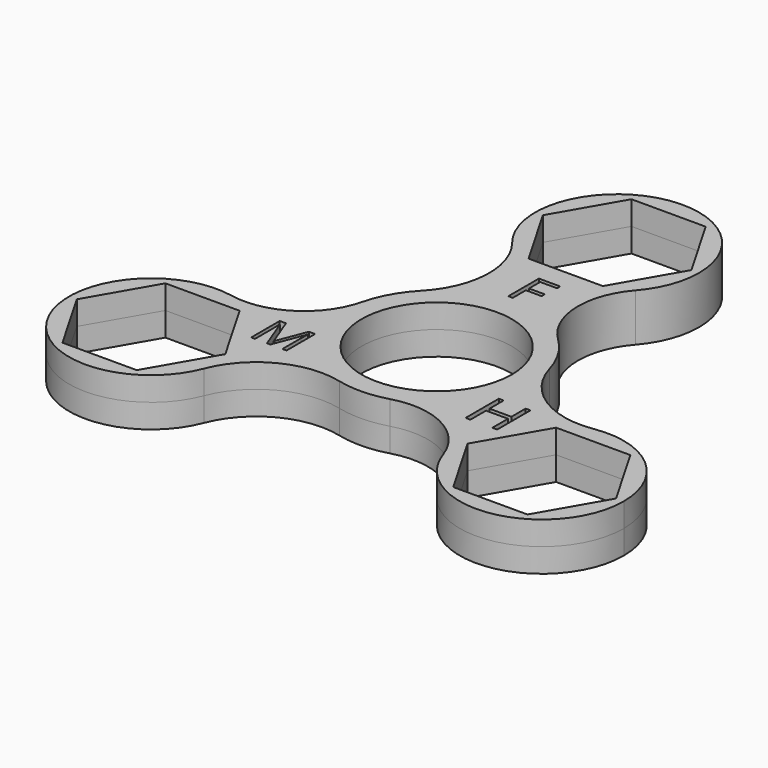
from build123d import *

# Parameters (mm, degrees)
F0_R           = 11
F1_DEPTH       = 3.5
F2_TEXT_SIZE   = 7.8320322144
F2_TEXT_SIZE_2 = 7.3181788644
F2_TEXT_SIZE_3 = 8.5313190033
F3_DEPTH       = 25


# Not quite as in the source:
# - Text() gives the source's letters only with a copy of the font that has no kerning and outlines rounded to 1/6400 em; it was checked with that copy


with BuildPart() as f1:
    # F0 (on Top) → F1 (new body, symmetric)
    with BuildSketch(Plane.XY):
        with BuildLine():
            ThreePointArc((-10.0686173445, 9.7274325889), (-0.2691708914, 13.9974121548), (9.6871937816, 10.1073377621))
            ThreePointArc((9.6871937816, 10.1073377621), (6.347333438, 17.4828570683), (9.0292648557, 25.1222415999))
            ThreePointArc((9.0292648557, 25.1222415999), (-0.2504407288, 21.0288021139), (-9.3512391392, 25.5059274026))
            ThreePointArc((-9.3512391392, 25.5059274026), (-6.7280894472, 17.4811090057), (-10.0686173445, 9.7274325889))
        make_face()
        with BuildLine():
            ThreePointArc((3.9096143758, -13.4430247873), (11.1967540221, -8.4043262293), (14, 0))
            ThreePointArc((14, 0), (13.863967212, 1.9468983398), (13.4585124078, 3.8559621069))
            ThreePointArc((13.4585124078, 3.8559621069), (11.9875290676, 7.2318149073), (9.6871937816, 10.1073377621))
            ThreePointArc((9.6871937816, 10.1073377621), (-0.2691708914, 13.9974121548), (-10.0686173445, 9.7274325889))
            ThreePointArc((-10.0686173445, 9.7274325889), (-12.256699959, 6.7655972475), (-13.5968081574, 3.3356870252))
            ThreePointArc((-13.5968081574, 3.3356870252), (-11.9875290676, -7.2318149073), (-3.3898950633, -13.5833946957))
            ThreePointArc((-3.3898950633, -13.5833946957), (0.2691708914, -13.9974121548), (3.9096143758, -13.4430247873))
        make_face()
        Circle(F0_R, mode=Mode.SUBTRACT)
        with BuildLine():
            ThreePointArc((-17.4131615082, -20.8513743528), (-11.7750397617, -14.567250883), (-3.3898950633, -13.5833946957))
            ThreePointArc((-3.3898950633, -13.5833946957), (-11.9875290676, -7.2318149073), (-13.5968081574, 3.3356870252))
            ThreePointArc((-13.5968081574, 3.3356870252), (-18.3142650709, -3.2444765306), (-26.2711318534, -4.7415480575))
            ThreePointArc((-26.2711318534, -4.7415480575), (-19.3288531038, -8.8961603469), (-16.6015182075, -16.5130942363))
            ThreePointArc((-16.6015182075, -16.5130942363), (-16.8061742025, -18.7198701207), (-17.4131615082, -20.8513743528))
        make_face()
        with BuildLine():
            ThreePointArc((13.4585124078, 3.8559621069), (13.863967212, 1.9468983398), (14, 0))
            ThreePointArc((14, 0), (11.1967540221, -8.4043262293), (3.9096143758, -13.4430247873))
            ThreePointArc((3.9096143758, -13.4430247873), (11.9669316329, -14.2383805377), (17.2418669977, -20.3806935425))
            ThreePointArc((17.2418669977, -20.3806935425), (18.3366972061, -10.2975130237), (26.7644006474, -4.6545530499))
            ThreePointArc((26.7644006474, -4.6545530499), (18.5031292089, -2.9138581227), (13.4585124078, 3.8559621069))
        make_face()
        with BuildLine():
            ThreePointArc((-9.3512391392, 25.5059274026), (-0.2504407288, 21.0288021139), (9.0292648557, 25.1222415999))
            ThreePointArc((9.0292648557, 25.1222415999), (11.232790799, 28.8042918768), (12, 33.0261884726))
            ThreePointArc((12, 33.0261884726), (-3.9865480261, 44.3446439695), (-9.3512391392, 25.5059274026))
        make_face()
        Polygon((10.8715055688, 33.0261884726), (5.4357527844, 23.6111884726), (-5.4357527844, 23.6111884726), (-10.8715055688, 33.0261884726), (-5.4357527844, 42.4411884726), (5.4357527844, 42.4411884726), align=None, mode=Mode.SUBTRACT)
        with BuildLine():
            ThreePointArc((-26.2711318534, -4.7415480575), (-39.1167799376, -22.2948993824), (-17.4131615082, -20.8513743528))
            ThreePointArc((-17.4131615082, -20.8513743528), (-16.8061742025, -18.7198701207), (-16.6015182075, -16.5130942363))
            ThreePointArc((-16.6015182075, -16.5130942363), (-19.3288531038, -8.8961603469), (-26.2711318534, -4.7415480575))
        make_face()
        Polygon((-23.1657654231, -25.9280942363), (-34.0372709919, -25.9280942363), (-39.4730237763, -16.5130942363), (-34.0372709919, -7.0980942363), (-23.1657654231, -7.0980942363), (-17.7300126386, -16.5130942363), align=None, mode=Mode.SUBTRACT)
        with BuildLine():
            ThreePointArc((40.6015182075, -16.5130942363), (36.4103141863, -7.4014146238), (26.7644006474, -4.6545530499))
            ThreePointArc((26.7644006474, -4.6545530499), (18.3366972061, -10.2975130237), (17.2418669977, -20.3806935425))
            ThreePointArc((17.2418669977, -20.3806935425), (30.5616439028, -28.3519247216), (40.6015182075, -16.5130942363))
        make_face()
        Polygon((34.0372709919, -7.0980942363), (39.4730237763, -16.5130942363), (34.0372709919, -25.9280942363), (23.1657654231, -25.9280942363), (17.7300126386, -16.5130942363), (23.1657654231, -7.0980942363), align=None, mode=Mode.SUBTRACT)
    extrude(amount=F1_DEPTH, both=True)

    # F2 (on face) → F3 (cut)
    with BuildSketch(Plane.XY.offset(3.5)):
        with Locations((-2.1966402851, 14.9032361805)):
            Text('F', F2_TEXT_SIZE, font='Open Sans', text_align=(TextAlign.LEFT, TextAlign.BOTTOM))
        with Locations((-18.7223702669, -11.4329964854)):
            Text('M', F2_TEXT_SIZE_2, font='Open Sans', text_align=(TextAlign.LEFT, TextAlign.BOTTOM))
        with Locations((12.7382390201, -11.6809140891)):
            Text('H', F2_TEXT_SIZE_3, font='Open Sans', text_align=(TextAlign.LEFT, TextAlign.BOTTOM))
    extrude(amount=-F3_DEPTH, mode=Mode.SUBTRACT)


solid = f1.part
